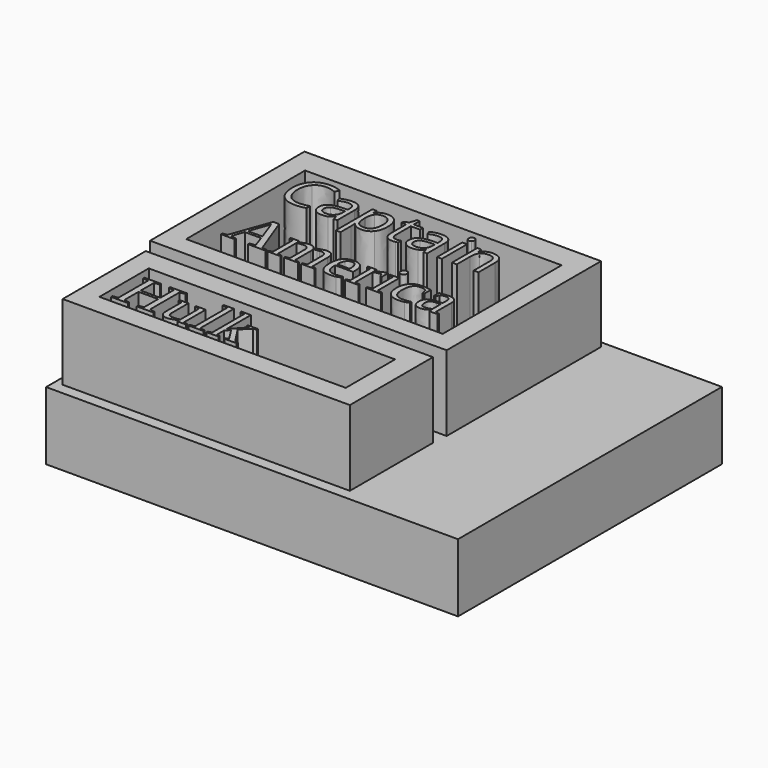
from build123d import *

# Parameters (mm, degrees)
F0_W          = 138.5813653469
F0_H          = 110.9895631671
F1_DEPTH      = 22.8698384017
F3_DEPTH      = 25.4
F4_DEPTH      = 25.4
F5_DEPTH      = 25.4
F6_DEPTH      = 25.4
F7_DEPTH      = 25.4
F2_W          = 1.612249592
F2_H          = 10.6396047259
F8_DEPTH      = 25.4
F9_DEPTH      = 25.4
F10_DEPTH     = 25.4
F11_DEPTH     = 25.4
F12_W         = 99.7868776321
F12_H         = 64.9340823293
F12_W_2       = 86.3021612167
F12_H_2       = 49.9971657991
F13_DEPTH     = 25.4
F14_W         = 96.6105125844
F14_H         = 34.9357193336
F14_W_2       = 82.8725360334
F14_H_2       = 20.7511782646
F15_DEPTH     = 25.4
F16_TEXT_SIZE = 21.4265555971
F17_DEPTH     = 25.4


# Not quite as in the source:
# - Text() gives the source's letters only with a copy of the font that has no kerning and outlines rounded to 1/6400 em; it was checked with that copy


with BuildPart() as f1:
    # F0 (on Top) → F1 (new body)
    with BuildSketch(Plane.XY):
        with Locations((2.9043704271, 4.875253886)):
            Rectangle(F0_W, F0_H)
    extrude(amount=F1_DEPTH)

    # F2 (on face) → F3 (join)
    with BuildSketch(Plane.XY.offset(22.8698384017)):
        with BuildLine():
            add(Edge.make_bspline(
                [(-49.4385806249, 46.1128756853), (-51.7777404376, 46.1128756853), (-53.1321543531, 44.5549890371)],
                knots=[0, 0, 0, 1, 1, 1], degree=2))
            add(Edge.make_bspline(
                [(-46.2140814408, 45.3580073792), (-47.8263310328, 46.1128756853), (-49.4385806249, 46.1128756853)],
                knots=[0, 0, 0, 1, 1, 1], degree=2))
            Line((-46.2140814408, 45.3580073792), (-45.5151293055, 46.7745503734))
            add(Edge.make_bspline(
                [(-49.4168354473, 47.5884413043), (-47.1864015223, 47.5884413043), (-45.5151293055, 46.7745503734)],
                knots=[0, 0, 0, 1, 1, 1], degree=2))
            add(Edge.make_bspline(
                [(-53.0622591396, 46.6953357981), (-51.5136918532, 47.5884413043), (-49.4168354473, 47.5884413043)],
                knots=[0, 0, 0, 1, 1, 1], degree=2))
            add(Edge.make_bspline(
                [(-55.4309302647, 44.1527032526), (-54.6108264259, 45.8022302919), (-53.0622591396, 46.6953357981)],
                knots=[0, 0, 0, 1, 1, 1], degree=2))
            add(Edge.make_bspline(
                [(-56.2510341034, 40.3100197355), (-56.2510341034, 42.5031762134), (-55.4309302647, 44.1527032526)],
                knots=[0, 0, 0, 1, 1, 1], degree=2))
            add(Edge.make_bspline(
                [(-54.5471441203, 34.9016834354), (-56.2510341034, 36.8059396973), (-56.2510341034, 40.3100197355)],
                knots=[0, 0, 0, 1, 1, 1], degree=2))
            add(Edge.make_bspline(
                [(-49.7088421172, 32.9974271735), (-52.8432541372, 32.9974271735), (-54.5471441203, 34.9016834354)],
                knots=[0, 0, 0, 1, 1, 1], degree=2))
            add(Edge.make_bspline(
                [(-46.0680781058, 33.5534824278), (-47.5436437248, 32.9974271735), (-49.7088421172, 32.9974271735)],
                knots=[0, 0, 0, 1, 1, 1], degree=2))
            Line((-46.0680781058, 33.5534824278), (-46.0680781058, 34.9979835074))
            add(Edge.make_bspline(
                [(-49.4572193485, 34.4636734307), (-47.9723343677, 34.4636734307), (-46.0680781058, 34.9979835074)],
                knots=[0, 0, 0, 1, 1, 1], degree=2))
            add(Edge.make_bspline(
                [(-53.1803043891, 35.9842826316), (-51.8740405096, 34.4636734307), (-49.4572193485, 34.4636734307)],
                knots=[0, 0, 0, 1, 1, 1], degree=2))
            add(Edge.make_bspline(
                [(-54.4865682686, 40.288274558), (-54.4865682686, 37.5048918326), (-53.1803043891, 35.9842826316)],
                knots=[0, 0, 0, 1, 1, 1], degree=2))
            add(Edge.make_bspline(
                [(-53.1321543531, 44.5549890371), (-54.4865682686, 42.997102389), (-54.4865682686, 40.288274558)],
                knots=[0, 0, 0, 1, 1, 1], degree=2))
        make_face()
        with BuildLine():
            add(Edge.make_bspline(
                [(-2.069186264, 20.8664472448), (-2.069186264, 20.406691862), (-2.4023423385, 20.0735357875)],
                knots=[0, 0, 0, 1, 1, 1], degree=2))
            add(Edge.make_bspline(
                [(-2.4023423385, 21.6693533843), (-2.069186264, 21.3361973098), (-2.069186264, 20.8664472448)],
                knots=[0, 0, 0, 1, 1, 1], degree=2))
            add(Edge.make_bspline(
                [(-3.2019169173, 22.0025094588), (-2.735498413, 22.0025094588), (-2.4023423385, 21.6693533843)],
                knots=[0, 0, 0, 1, 1, 1], degree=2))
            add(Edge.make_bspline(
                [(-3.9948283746, 21.6693533843), (-3.6616723001, 22.0025094588), (-3.2019169173, 22.0025094588)],
                knots=[0, 0, 0, 1, 1, 1], degree=2))
            add(Edge.make_bspline(
                [(-4.3279844491, 20.8664472448), (-4.3279844491, 21.3361973098), (-3.9948283746, 21.6693533843)],
                knots=[0, 0, 0, 1, 1, 1], degree=2))
            add(Edge.make_bspline(
                [(-3.9948283746, 20.0735357875), (-4.3279844491, 20.406691862), (-4.3279844491, 20.8664472448)],
                knots=[0, 0, 0, 1, 1, 1], degree=2))
            add(Edge.make_bspline(
                [(-3.2019169173, 19.740379713), (-3.6616723001, 19.740379713), (-3.9948283746, 20.0735357875)],
                knots=[0, 0, 0, 1, 1, 1], degree=2))
            add(Edge.make_bspline(
                [(-2.4023423385, 20.0735357875), (-2.735498413, 19.740379713), (-3.2019169173, 19.740379713)],
                knots=[0, 0, 0, 1, 1, 1], degree=2))
        make_face()
    extrude(amount=F3_DEPTH)

    # F2 (on face) → F4 (join)
    with BuildSketch(Plane.XY.offset(22.8698384017)):
        with BuildLine():
            Line((-36.991019709, 34.7090832915), (-36.6710549537, 33.1931337714))
            Line((-36.6710549537, 33.1931337714), (-35.4750701889, 33.1931337714))
            Line((-35.4750701889, 33.1931337714), (-35.4750701889, 40.4560230705))
            add(Edge.make_bspline(
                [(-36.3930273266, 43.1632976745), (-35.4750701889, 42.3198954312), (-35.4750701889, 40.4560230705)],
                knots=[0, 0, 0, 1, 1, 1], degree=2))
            add(Edge.make_bspline(
                [(-39.2121342722, 44.0066999177), (-37.3109844643, 44.0066999177), (-36.3930273266, 43.1632976745)],
                knots=[0, 0, 0, 1, 1, 1], degree=2))
            add(Edge.make_bspline(
                [(-41.0930921296, 43.7643965108), (-40.1564962683, 44.0066999177), (-39.2121342722, 44.0066999177)],
                knots=[0, 0, 0, 1, 1, 1], degree=2))
            add(Edge.make_bspline(
                [(-42.8156208363, 43.0965089149), (-42.0296879909, 43.5220931039), (-41.0930921296, 43.7643965108)],
                knots=[0, 0, 0, 1, 1, 1], degree=2))
            Line((-42.8156208363, 43.0965089149), (-42.3185882068, 41.8632467028))
            add(Edge.make_bspline(
                [(-39.3115407981, 42.6771376337), (-40.6411030821, 42.6771376337), (-42.3185882068, 41.8632467028)],
                knots=[0, 0, 0, 1, 1, 1], degree=2))
            add(Edge.make_bspline(
                [(-37.5874588644, 42.0806984783), (-38.1248753951, 42.6771376337), (-39.3115407981, 42.6771376337)],
                knots=[0, 0, 0, 1, 1, 1], degree=2))
            add(Edge.make_bspline(
                [(-37.0500423338, 40.2323583872), (-37.0500423338, 41.4842593228), (-37.5874588644, 42.0806984783)],
                knots=[0, 0, 0, 1, 1, 1], degree=2))
            Line((-37.0500423338, 40.2323583872), (-37.0500423338, 39.5706836991))
            Line((-37.0500423338, 39.5706836991), (-38.8548920697, 39.5116610744))
            add(Edge.make_bspline(
                [(-44.0084991472, 36.1349456475), (-44.0084991472, 39.3563383776), (-38.8548920697, 39.5116610744)],
                knots=[0, 0, 0, 1, 1, 1], degree=2))
            add(Edge.make_bspline(
                [(-43.1107339601, 33.8144245583), (-44.0084991472, 34.6314219431), (-44.0084991472, 36.1349456475)],
                knots=[0, 0, 0, 1, 1, 1], degree=2))
            add(Edge.make_bspline(
                [(-40.6317837203, 32.9974271735), (-42.212968773, 32.9974271735), (-43.1107339601, 33.8144245583)],
                knots=[0, 0, 0, 1, 1, 1], degree=2))
            add(Edge.make_bspline(
                [(-38.654525791, 33.3531161491), (-39.4451183173, 32.9974271735), (-40.6317837203, 32.9974271735)],
                knots=[0, 0, 0, 1, 1, 1], degree=2))
            add(Edge.make_bspline(
                [(-37.0686810574, 34.7090832915), (-37.8639332646, 33.7088051246), (-38.654525791, 33.3531161491)],
                knots=[0, 0, 0, 1, 1, 1], degree=2))
            Line((-37.0686810574, 34.7090832915), (-36.991019709, 34.7090832915))
        make_face()
        with BuildLine():
            add(Edge.make_bspline(
                [(-40.3118189651, 34.3300959115), (-38.8051888068, 34.3300959115), (-37.9462542939, 35.1548594311)],
                knots=[0, 0, 0, 1, 1, 1], degree=2))
            add(Edge.make_bspline(
                [(-41.7904910379, 34.7851914129), (-41.262393869, 34.3300959115), (-40.3118189651, 34.3300959115)],
                knots=[0, 0, 0, 1, 1, 1], degree=2))
            add(Edge.make_bspline(
                [(-42.3185882068, 36.1163069239), (-42.3185882068, 35.2402869143), (-41.7904910379, 34.7851914129)],
                knots=[0, 0, 0, 1, 1, 1], degree=2))
            add(Edge.make_bspline(
                [(-41.4705262827, 37.7611742822), (-42.3185882068, 37.2315238864), (-42.3185882068, 36.1163069239)],
                knots=[0, 0, 0, 1, 1, 1], degree=2))
            add(Edge.make_bspline(
                [(-38.699569373, 38.3591666646), (-40.6224643585, 38.2908246781), (-41.4705262827, 37.7611742822)],
                knots=[0, 0, 0, 1, 1, 1], degree=2))
            Line((-38.699569373, 38.3591666646), (-37.087319781, 38.4244021973))
            Line((-37.087319781, 38.4244021973), (-37.087319781, 37.4645079315))
            add(Edge.make_bspline(
                [(-37.9462542939, 35.1548594311), (-37.087319781, 35.9796229507), (-37.087319781, 37.4645079315)],
                knots=[0, 0, 0, 1, 1, 1], degree=2))
        make_face(mode=Mode.SUBTRACT)
    extrude(amount=F4_DEPTH)

    # F2 (on face) → F5 (join)
    with BuildSketch(Plane.XY.offset(22.8698384017)):
        with BuildLine():
            add(Edge.make_bspline(
                [(-27.2056898151, 32.9974271735), (-28.2463518832, 32.9974271735), (-29.1052863961, 33.3810742345)],
                knots=[0, 0, 0, 1, 1, 1], degree=2))
            add(Edge.make_bspline(
                [(-23.9578922265, 34.449694388), (-25.1274721328, 32.9974271735), (-27.2056898151, 32.9974271735)],
                knots=[0, 0, 0, 1, 1, 1], degree=2))
            add(Edge.make_bspline(
                [(-22.7883123201, 38.5238087232), (-22.7883123201, 35.9019616024), (-23.9578922265, 34.449694388)],
                knots=[0, 0, 0, 1, 1, 1], degree=2))
            add(Edge.make_bspline(
                [(-23.9392535029, 42.5808375617), (-22.7883123201, 41.1332300282), (-22.7883123201, 38.5238087232)],
                knots=[0, 0, 0, 1, 1, 1], degree=2))
            add(Edge.make_bspline(
                [(-27.2056898151, 44.0284450952), (-25.0901946856, 44.0284450952), (-23.9392535029, 42.5808375617)],
                knots=[0, 0, 0, 1, 1, 1], degree=2))
            add(Edge.make_bspline(
                [(-29.0990734882, 43.6401383534), (-28.2743099686, 44.0284450952), (-27.2056898151, 44.0284450952)],
                knots=[0, 0, 0, 1, 1, 1], degree=2))
            add(Edge.make_bspline(
                [(-30.5451277947, 42.375811602), (-29.9238370078, 43.2518316116), (-29.0990734882, 43.6401383534)],
                knots=[0, 0, 0, 1, 1, 1], degree=2))
            Line((-30.5451277947, 42.375811602), (-30.6227891431, 42.375811602))
            Line((-30.6227891431, 42.375811602), (-30.8464538264, 43.8327384974))
            Line((-30.8464538264, 43.8327384974), (-32.1573773868, 43.8327384974))
            Line((-32.1573773868, 43.8327384974), (-32.1573773868, 28.41540762))
            Line((-32.1573773868, 28.41540762), (-30.5451277947, 28.41540762))
            Line((-30.5451277947, 28.41540762), (-30.5451277947, 32.7955076678))
            add(Edge.make_bspline(
                [(-30.6631730443, 34.5630799566), (-30.5451277947, 33.6311437762), (-30.5451277947, 32.7955076678)],
                knots=[0, 0, 0, 1, 1, 1], degree=2))
            Line((-30.6631730443, 34.5630799566), (-30.5451277947, 34.5630799566))
            add(Edge.make_bspline(
                [(-29.1052863961, 33.3810742345), (-29.964220909, 33.7647212954), (-30.5451277947, 34.5630799566)],
                knots=[0, 0, 0, 1, 1, 1], degree=2))
        make_face()
        with BuildLine():
            add(Edge.make_bspline(
                [(-27.4386738602, 42.6584989101), (-29.0695621758, 42.6584989101), (-29.7980256235, 41.7560740421)],
                knots=[0, 0, 0, 1, 1, 1], degree=2))
            add(Edge.make_bspline(
                [(-25.2408577014, 41.5960916645), (-26.022130866, 42.6584989101), (-27.4386738602, 42.6584989101)],
                knots=[0, 0, 0, 1, 1, 1], degree=2))
            add(Edge.make_bspline(
                [(-24.4595845369, 38.5424474468), (-24.4595845369, 40.5336844188), (-25.2408577014, 41.5960916645)],
                knots=[0, 0, 0, 1, 1, 1], degree=2))
            add(Edge.make_bspline(
                [(-25.2408577014, 35.4655048246), (-24.4595845369, 36.582275014), (-24.4595845369, 38.5424474468)],
                knots=[0, 0, 0, 1, 1, 1], degree=2))
            add(Edge.make_bspline(
                [(-27.4013964129, 34.3487346351), (-26.022130866, 34.3487346351), (-25.2408577014, 35.4655048246)],
                knots=[0, 0, 0, 1, 1, 1], degree=2))
            add(Edge.make_bspline(
                [(-29.7980256235, 35.3148418087), (-29.0509234522, 34.3487346351), (-27.4013964129, 34.3487346351)],
                knots=[0, 0, 0, 1, 1, 1], degree=2))
            add(Edge.make_bspline(
                [(-30.5451277947, 38.5238087232), (-30.5451277947, 36.2809489824), (-29.7980256235, 35.3148418087)],
                knots=[0, 0, 0, 1, 1, 1], degree=2))
            Line((-30.5451277947, 38.5238087232), (-30.5451277947, 38.8810509256))
            add(Edge.make_bspline(
                [(-29.7980256235, 41.7560740421), (-30.5264890711, 40.8536491741), (-30.5451277947, 38.8810509256)],
                knots=[0, 0, 0, 1, 1, 1], degree=2))
        make_face(mode=Mode.SUBTRACT)
    extrude(amount=F5_DEPTH)

    # F2 (on face) → F6 (join)
    with BuildSketch(Plane.XY.offset(22.8698384017)):
        with BuildLine():
            add(Edge.make_bspline(
                [(-16.5381270037, 34.3300959115), (-16.1094363607, 34.3300959115), (-15.7118102571, 34.3922249902)],
                knots=[0, 0, 0, 1, 1, 1], degree=2))
            add(Edge.make_bspline(
                [(-17.7900279394, 34.8442140376), (-17.333379211, 34.3300959115), (-16.5381270037, 34.3300959115)],
                knots=[0, 0, 0, 1, 1, 1], degree=2))
            add(Edge.make_bspline(
                [(-18.2466766677, 36.3182264296), (-18.2466766677, 35.3583321638), (-17.7900279394, 34.8442140376)],
                knots=[0, 0, 0, 1, 1, 1], degree=2))
            Line((-18.2466766677, 36.3182264296), (-18.2466766677, 42.5808375617))
            Line((-18.2466766677, 42.5808375617), (-15.1588614568, 42.5808375617))
            Line((-15.1588614568, 42.5808375617), (-15.1588614568, 43.8327384974))
            Line((-15.1588614568, 43.8327384974), (-18.2466766677, 43.8327384974))
            Line((-18.2466766677, 43.8327384974), (-18.2466766677, 46.2992629214))
            Line((-18.2466766677, 46.2992629214), (-19.1786128481, 46.2992629214))
            Line((-19.1786128481, 46.2992629214), (-19.8558198058, 44.0284450952))
            Line((-19.8558198058, 44.0284450952), (-21.3810886877, 43.3574510454))
            Line((-21.3810886877, 43.3574510454), (-21.3810886877, 42.5808375617))
            Line((-21.3810886877, 42.5808375617), (-19.8558198058, 42.5808375617))
            Line((-19.8558198058, 42.5808375617), (-19.8558198058, 36.249884443))
            add(Edge.make_bspline(
                [(-16.7711110488, 32.9974271735), (-19.8558198058, 32.9974271735), (-19.8558198058, 36.249884443)],
                knots=[0, 0, 0, 1, 1, 1], degree=2))
            add(Edge.make_bspline(
                [(-15.8516006842, 33.0813014298), (-16.3610591294, 32.9974271735), (-16.7711110488, 32.9974271735)],
                knots=[0, 0, 0, 1, 1, 1], degree=2))
            add(Edge.make_bspline(
                [(-15.0812001084, 33.2894338434), (-15.3421422389, 33.165175686), (-15.8516006842, 33.0813014298)],
                knots=[0, 0, 0, 1, 1, 1], degree=2))
            Line((-15.0812001084, 33.2894338434), (-15.0812001084, 34.5226960554))
            add(Edge.make_bspline(
                [(-15.7118102571, 34.3922249902), (-15.3141841535, 34.4543540689), (-15.0812001084, 34.5226960554)],
                knots=[0, 0, 0, 1, 1, 1], degree=2))
        make_face()
    extrude(amount=F6_DEPTH)

    # F2 (on face) → F7 (join)
    with BuildSketch(Plane.XY.offset(22.8698384017)):
        with BuildLine():
            Line((-6.7341583862, 34.7090832915), (-6.4141936309, 33.1931337714))
            Line((-6.4141936309, 33.1931337714), (-5.2182088661, 33.1931337714))
            Line((-5.2182088661, 33.1931337714), (-5.2182088661, 40.4560230705))
            add(Edge.make_bspline(
                [(-6.1361660038, 43.1632976745), (-5.2182088661, 42.3198954312), (-5.2182088661, 40.4560230705)],
                knots=[0, 0, 0, 1, 1, 1], degree=2))
            add(Edge.make_bspline(
                [(-8.9552729494, 44.0066999177), (-7.0541231414, 44.0066999177), (-6.1361660038, 43.1632976745)],
                knots=[0, 0, 0, 1, 1, 1], degree=2))
            add(Edge.make_bspline(
                [(-10.8362308068, 43.7643965108), (-9.8996349455, 44.0066999177), (-8.9552729494, 44.0066999177)],
                knots=[0, 0, 0, 1, 1, 1], degree=2))
            add(Edge.make_bspline(
                [(-12.5587595135, 43.0965089149), (-11.7728266681, 43.5220931039), (-10.8362308068, 43.7643965108)],
                knots=[0, 0, 0, 1, 1, 1], degree=2))
            Line((-12.5587595135, 43.0965089149), (-12.061726884, 41.8632467028))
            add(Edge.make_bspline(
                [(-9.0546794753, 42.6771376337), (-10.3842417593, 42.6771376337), (-12.061726884, 41.8632467028)],
                knots=[0, 0, 0, 1, 1, 1], degree=2))
            add(Edge.make_bspline(
                [(-7.3305975416, 42.0806984783), (-7.8680140723, 42.6771376337), (-9.0546794753, 42.6771376337)],
                knots=[0, 0, 0, 1, 1, 1], degree=2))
            add(Edge.make_bspline(
                [(-6.7931810109, 40.2323583872), (-6.7931810109, 41.4842593228), (-7.3305975416, 42.0806984783)],
                knots=[0, 0, 0, 1, 1, 1], degree=2))
            Line((-6.7931810109, 40.2323583872), (-6.7931810109, 39.5706836991))
            Line((-6.7931810109, 39.5706836991), (-8.5980307469, 39.5116610744))
            add(Edge.make_bspline(
                [(-13.7516378244, 36.1349456475), (-13.7516378244, 39.3563383776), (-8.5980307469, 39.5116610744)],
                knots=[0, 0, 0, 1, 1, 1], degree=2))
            add(Edge.make_bspline(
                [(-12.8538726373, 33.8144245583), (-13.7516378244, 34.6314219431), (-13.7516378244, 36.1349456475)],
                knots=[0, 0, 0, 1, 1, 1], degree=2))
            add(Edge.make_bspline(
                [(-10.3749223975, 32.9974271735), (-11.9561074502, 32.9974271735), (-12.8538726373, 33.8144245583)],
                knots=[0, 0, 0, 1, 1, 1], degree=2))
            add(Edge.make_bspline(
                [(-8.3976644681, 33.3531161491), (-9.1882569945, 32.9974271735), (-10.3749223975, 32.9974271735)],
                knots=[0, 0, 0, 1, 1, 1], degree=2))
            add(Edge.make_bspline(
                [(-6.8118197345, 34.7090832915), (-7.6070719418, 33.7088051246), (-8.3976644681, 33.3531161491)],
                knots=[0, 0, 0, 1, 1, 1], degree=2))
            Line((-6.8118197345, 34.7090832915), (-6.7341583862, 34.7090832915))
        make_face()
        with BuildLine():
            add(Edge.make_bspline(
                [(-10.0549576422, 34.3300959115), (-8.548327484, 34.3300959115), (-7.6893929711, 35.1548594311)],
                knots=[0, 0, 0, 1, 1, 1], degree=2))
            add(Edge.make_bspline(
                [(-11.5336297151, 34.7851914129), (-11.0055325462, 34.3300959115), (-10.0549576422, 34.3300959115)],
                knots=[0, 0, 0, 1, 1, 1], degree=2))
            add(Edge.make_bspline(
                [(-12.061726884, 36.1163069239), (-12.061726884, 35.2402869143), (-11.5336297151, 34.7851914129)],
                knots=[0, 0, 0, 1, 1, 1], degree=2))
            add(Edge.make_bspline(
                [(-11.2136649598, 37.7611742822), (-12.061726884, 37.2315238864), (-12.061726884, 36.1163069239)],
                knots=[0, 0, 0, 1, 1, 1], degree=2))
            add(Edge.make_bspline(
                [(-8.4427080502, 38.3591666646), (-10.3656030357, 38.2908246781), (-11.2136649598, 37.7611742822)],
                knots=[0, 0, 0, 1, 1, 1], degree=2))
            Line((-8.4427080502, 38.3591666646), (-6.8304584582, 38.4244021973))
            Line((-6.8304584582, 38.4244021973), (-6.8304584582, 37.4645079315))
            add(Edge.make_bspline(
                [(-7.6893929711, 35.1548594311), (-6.8304584582, 35.9796229507), (-6.8304584582, 37.4645079315)],
                knots=[0, 0, 0, 1, 1, 1], degree=2))
        make_face(mode=Mode.SUBTRACT)
    extrude(amount=F7_DEPTH)

    # F2 (on face) → F8 (join)
    with BuildSketch(Plane.XY.offset(22.8698384017)):
        with BuildLine():
            add(Edge.make_bspline(
                [(-2.0372000371, 46.7155277487), (-2.0372000371, 47.268476549), (-1.7653853178, 47.5263122256)],
                knots=[0, 0, 0, 1, 1, 1], degree=2))
            add(Edge.make_bspline(
                [(-1.7653853178, 45.9047432717), (-2.0372000371, 46.1718983101), (-2.0372000371, 46.7155277487)],
                knots=[0, 0, 0, 1, 1, 1], degree=2))
            add(Edge.make_bspline(
                [(-1.0835186792, 45.6375882334), (-1.4935705985, 45.6375882334), (-1.7653853178, 45.9047432717)],
                knots=[0, 0, 0, 1, 1, 1], degree=2))
            add(Edge.make_bspline(
                [(-0.4140778563, 45.9047432717), (-0.6952119374, 45.6375882334), (-1.0835186792, 45.6375882334)],
                knots=[0, 0, 0, 1, 1, 1], degree=2))
            add(Edge.make_bspline(
                [(-0.1329437752, 46.7155277487), (-0.1329437752, 46.1718983101), (-0.4140778563, 45.9047432717)],
                knots=[0, 0, 0, 1, 1, 1], degree=2))
            add(Edge.make_bspline(
                [(-0.4140778563, 47.5216525447), (-0.1329437752, 47.2591571872), (-0.1329437752, 46.7155277487)],
                knots=[0, 0, 0, 1, 1, 1], degree=2))
            add(Edge.make_bspline(
                [(-1.0835186792, 47.7841479021), (-0.6952119374, 47.7841479021), (-0.4140778563, 47.5216525447)],
                knots=[0, 0, 0, 1, 1, 1], degree=2))
            add(Edge.make_bspline(
                [(-1.7653853178, 47.5263122256), (-1.4935705985, 47.7841479021), (-1.0835186792, 47.7841479021)],
                knots=[0, 0, 0, 1, 1, 1], degree=2))
        make_face()
        with Locations((-1.0943912679, 38.5129361344)):
            Rectangle(F2_W, F2_H)
    extrude(amount=F8_DEPTH)

    # F2 (on face) → F9 (join)
    with BuildSketch(Plane.XY.offset(22.8698384017)):
        with BuildLine():
            Line((10.4103608788, 40.0770356905), (10.4103608788, 33.1931337714))
            Line((10.4103608788, 33.1931337714), (12.0226104708, 33.1931337714))
            Line((12.0226104708, 33.1931337714), (12.0226104708, 40.1329518613))
            add(Edge.make_bspline(
                [(11.0518436163, 43.1011685958), (12.0226104708, 42.1738920963), (12.0226104708, 40.1329518613)],
                knots=[0, 0, 0, 1, 1, 1], degree=2))
            add(Edge.make_bspline(
                [(8.1581817762, 44.0284450952), (10.0810767617, 44.0284450952), (11.0518436163, 43.1011685958)],
                knots=[0, 0, 0, 1, 1, 1], degree=2))
            add(Edge.make_bspline(
                [(6.1684980311, 43.5950947714), (7.0616035373, 44.0284450952), (8.1581817762, 44.0284450952)],
                knots=[0, 0, 0, 1, 1, 1], degree=2))
            add(Edge.make_bspline(
                [(4.7783598954, 42.375811602), (5.2753925249, 43.1617444475), (6.1684980311, 43.5950947714)],
                knots=[0, 0, 0, 1, 1, 1], degree=2))
            Line((4.7783598954, 42.375811602), (4.700698547, 42.375811602))
            Line((4.700698547, 42.375811602), (4.4397564165, 43.8327384974))
            Line((4.4397564165, 43.8327384974), (3.1288328561, 43.8327384974))
            Line((3.1288328561, 43.8327384974), (3.1288328561, 33.1931337714))
            Line((3.1288328561, 33.1931337714), (4.7410824482, 33.1931337714))
            Line((4.7410824482, 33.1931337714), (4.7410824482, 38.7754314919))
            add(Edge.make_bspline(
                [(5.5176959318, 41.7560740421), (4.7410824482, 40.8536491741), (4.7410824482, 38.7754314919)],
                knots=[0, 0, 0, 1, 1, 1], degree=2))
            add(Edge.make_bspline(
                [(7.9624751783, 42.6584989101), (6.2943094155, 42.6584989101), (5.5176959318, 41.7560740421)],
                knots=[0, 0, 0, 1, 1, 1], degree=2))
            add(Edge.make_bspline(
                [(9.8185814042, 42.0170161726), (9.2268019297, 42.6584989101), (7.9624751783, 42.6584989101)],
                knots=[0, 0, 0, 1, 1, 1], degree=2))
            add(Edge.make_bspline(
                [(10.4103608788, 40.0770356905), (10.4103608788, 41.3755334351), (9.8185814042, 42.0170161726)],
                knots=[0, 0, 0, 1, 1, 1], degree=2))
        make_face()
    extrude(amount=F9_DEPTH)

    # F2 (on face) → F10 (join)
    with BuildSketch(Plane.XY.offset(22.8698384017)):
        Polygon((-49.7604783288, 7.8833550215), (-49.7604783288, 8.4363941051), (-51.6361470282, 8.7162452077), (-50.2302283939, 12.7441021484), (-44.7331531646, 12.7441021484), (-43.3472238947, 8.7162452077), (-45.2228925941, 8.4363941051), (-45.2228925941, 7.8833550215), (-39.319366954, 7.8833550215), (-39.319366954, 8.4363941051), (-41.0884257096, 8.7162452077), (-46.0357934159, 21.9591991691), (-48.0114089377, 21.9591991691), (-52.7688776816, 8.7162452077), (-54.3513690354, 8.4363941051), (-54.3513690354, 7.8833550215), align=None)
        Polygon((-49.9170616838, 13.6836022785), (-47.5216695082, 20.4599968339), (-45.0563145569, 13.6836022785), align=None, mode=Mode.SUBTRACT)
        with BuildLine():
            add(Edge.make_bspline(
                [(-35.7679231998, 16.878569033), (-34.9883379854, 17.3249981728), (-34.1138032899, 17.6281702006)],
                knots=[0, 0, 0, 1, 1, 1], degree=2))
            Line((-35.7679231998, 16.878569033), (-35.8512122184, 17.6714804903))
            Line((-35.8512122184, 17.6714804903), (-38.7163544591, 17.6714804903))
            Line((-38.7163544591, 17.6714804903), (-38.7163544591, 17.2017304253))
            Line((-38.7163544591, 17.2017304253), (-37.477013862, 16.9418686872))
            Line((-37.477013862, 16.9418686872), (-37.477013862, 8.6129668246))
            Line((-37.477013862, 8.6129668246), (-38.7163544591, 8.3531050865))
            Line((-38.7163544591, 8.3531050865), (-38.7163544591, 7.8833550215))
            Line((-38.7163544591, 7.8833550215), (-34.2787155468, 7.8833550215))
            Line((-34.2787155468, 7.8833550215), (-34.2787155468, 8.3531050865))
            Line((-34.2787155468, 8.3531050865), (-35.7479338353, 8.6129668246))
            Line((-35.7479338353, 8.6129668246), (-35.7479338353, 16.3488508745))
            add(Edge.make_bspline(
                [(-33.4691462857, 16.6486913416), (-34.3853254906, 16.6486913416), (-35.7479338353, 16.3488508745)],
                knots=[0, 0, 0, 1, 1, 1], degree=2))
            add(Edge.make_bspline(
                [(-32.1398535485, 16.185604398), (-32.5829511276, 16.6486913416), (-33.4691462857, 16.6486913416)],
                knots=[0, 0, 0, 1, 1, 1], degree=2))
            add(Edge.make_bspline(
                [(-31.6967559694, 14.8596432215), (-31.6967559694, 15.7225174545), (-32.1398535485, 16.185604398)],
                knots=[0, 0, 0, 1, 1, 1], degree=2))
            Line((-31.6967559694, 14.8596432215), (-31.6967559694, 8.6129668246))
            Line((-31.6967559694, 8.6129668246), (-33.1459848935, 8.3531050865))
            Line((-33.1459848935, 8.3531050865), (-33.1459848935, 7.8833550215))
            Line((-33.1459848935, 7.8833550215), (-28.5017892149, 7.8833550215))
            Line((-28.5017892149, 7.8833550215), (-28.5017892149, 8.3531050865))
            Line((-28.5017892149, 8.3531050865), (-29.9710075035, 8.6129668246))
            Line((-29.9710075035, 8.6129668246), (-29.9710075035, 15.0462106232))
            add(Edge.make_bspline(
                [(-30.147580223, 16.2855512204), (-29.9710075035, 15.7225174545), (-29.9710075035, 15.0462106232)],
                knots=[0, 0, 0, 1, 1, 1], degree=2))
            add(Edge.make_bspline(
                [(-29.5995384804, 16.3938269446), (-29.9276972138, 16.3255299493), (-30.147580223, 16.2855512204)],
                knots=[0, 0, 0, 1, 1, 1], degree=2))
            add(Edge.make_bspline(
                [(-28.9132369669, 16.5137631314), (-29.271379747, 16.4621239399), (-29.5995384804, 16.3938269446)],
                knots=[0, 0, 0, 1, 1, 1], degree=2))
            add(Edge.make_bspline(
                [(-28.1952856264, 16.6070468323), (-28.5550941868, 16.565402323), (-28.9132369669, 16.5137631314)],
                knots=[0, 0, 0, 1, 1, 1], degree=2))
            add(Edge.make_bspline(
                [(-27.5656206456, 16.6486913416), (-27.8354770659, 16.6486913416), (-28.1952856264, 16.6070468323)],
                knots=[0, 0, 0, 1, 1, 1], degree=2))
            add(Edge.make_bspline(
                [(-25.8998402731, 14.8596432215), (-25.8998402731, 16.6486913416), (-27.5656206456, 16.6486913416)],
                knots=[0, 0, 0, 1, 1, 1], degree=2))
            Line((-25.8998402731, 14.8596432215), (-25.8998402731, 8.6129668246))
            Line((-25.8998402731, 8.6129668246), (-27.3557323186, 8.3531050865))
            Line((-27.3557323186, 8.3531050865), (-27.3557323186, 7.8833550215))
            Line((-27.3557323186, 7.8833550215), (-22.9114302848, 7.8833550215))
            Line((-22.9114302848, 7.8833550215), (-22.9114302848, 8.3531050865))
            Line((-22.9114302848, 8.3531050865), (-24.1707602464, 8.6129668246))
            Line((-24.1707602464, 8.6129668246), (-24.1707602464, 15.0462106232))
            add(Edge.make_bspline(
                [(-26.6694308052, 17.9313422284), (-24.1707602464, 17.9313422284), (-24.1707602464, 15.0462106232)],
                knots=[0, 0, 0, 1, 1, 1], degree=2))
            add(Edge.make_bspline(
                [(-28.4534815841, 17.5865256913), (-27.3757216831, 17.9313422284), (-26.6694308052, 17.9313422284)],
                knots=[0, 0, 0, 1, 1, 1], degree=2))
            add(Edge.make_bspline(
                [(-30.3341476247, 16.7952800144), (-29.5312414851, 17.2417091542), (-28.4534815841, 17.5865256913)],
                knots=[0, 0, 0, 1, 1, 1], degree=2))
            add(Edge.make_bspline(
                [(-31.2453294884, 17.6598200277), (-30.6373196525, 17.388297827), (-30.3341476247, 16.7952800144)],
                knots=[0, 0, 0, 1, 1, 1], degree=2))
            add(Edge.make_bspline(
                [(-32.5729564453, 17.9313422284), (-31.8533393244, 17.9313422284), (-31.2453294884, 17.6598200277)],
                knots=[0, 0, 0, 1, 1, 1], degree=2))
            add(Edge.make_bspline(
                [(-34.1138032899, 17.6281702006), (-33.2392685943, 17.9313422284), (-32.5729564453, 17.9313422284)],
                knots=[0, 0, 0, 1, 1, 1], degree=2))
        make_face()
        with BuildLine():
            Line((-19.8697153246, 12.6208344009), (-19.8697153246, 12.8074018026))
            Line((-19.8697153246, 12.8074018026), (-13.8529166191, 12.8074018026))
            Line((-13.8529166191, 12.8074018026), (-13.8529166191, 13.6602813533))
            add(Edge.make_bspline(
                [(-17.6109171395, 17.9313422284), (-13.8529166191, 17.9313422284), (-13.8529166191, 13.6602813533)],
                knots=[0, 0, 0, 1, 1, 1], degree=2))
            add(Edge.make_bspline(
                [(-20.6726214641, 16.6703464864), (-19.5998589043, 17.9313422284), (-17.6109171395, 17.9313422284)],
                knots=[0, 0, 0, 1, 1, 1], degree=2))
            add(Edge.make_bspline(
                [(-21.745384024, 12.8507120923), (-21.745384024, 15.4093507444), (-20.6726214641, 16.6703464864)],
                knots=[0, 0, 0, 1, 1, 1], degree=2))
            add(Edge.make_bspline(
                [(-20.6892792679, 8.9028126094), (-21.745384024, 10.1321585244), (-21.745384024, 12.8507120923)],
                knots=[0, 0, 0, 1, 1, 1], degree=2))
            add(Edge.make_bspline(
                [(-17.3510554014, 7.6734666945), (-19.6331745117, 7.6734666945), (-20.6892792679, 8.9028126094)],
                knots=[0, 0, 0, 1, 1, 1], degree=2))
            add(Edge.make_bspline(
                [(-15.5969886691, 7.9133390682), (-16.454865561, 7.6734666945), (-17.3510554014, 7.6734666945)],
                knots=[0, 0, 0, 1, 1, 1], degree=2))
            add(Edge.make_bspline(
                [(-14.2393776655, 8.4763728341), (-14.7391117773, 8.1532114418), (-15.5969886691, 7.9133390682)],
                knots=[0, 0, 0, 1, 1, 1], degree=2))
            Line((-14.2393776655, 8.4763728341), (-14.2393776655, 9.0593959645))
            add(Edge.make_bspline(
                [(-15.5087023094, 8.8528391983), (-14.7391117773, 8.9461228991), (-14.2393776655, 9.0593959645)],
                knots=[0, 0, 0, 1, 1, 1], degree=2))
            add(Edge.make_bspline(
                [(-16.8413266074, 8.7595554974), (-16.2782928415, 8.7595554974), (-15.5087023094, 8.8528391983)],
                knots=[0, 0, 0, 1, 1, 1], degree=2))
            add(Edge.make_bspline(
                [(-18.5754039752, 9.1760005905), (-17.9140891673, 8.7595554974), (-16.8413266074, 8.7595554974)],
                knots=[0, 0, 0, 1, 1, 1], degree=2))
            add(Edge.make_bspline(
                [(-19.5532170538, 10.3886887017), (-19.2367187831, 9.5924456837), (-18.5754039752, 9.1760005905)],
                knots=[0, 0, 0, 1, 1, 1], degree=2))
            add(Edge.make_bspline(
                [(-19.8697153246, 12.6208344009), (-19.8697153246, 11.1849317198), (-19.5532170538, 10.3886887017)],
                knots=[0, 0, 0, 1, 1, 1], degree=2))
        make_face()
        with BuildLine():
            add(Edge.make_bspline(
                [(-17.6109171395, 17.0984520422), (-18.6936743816, 17.0984520422), (-19.2717001709, 16.2239173466)],
                knots=[0, 0, 0, 1, 1, 1], degree=2))
            add(Edge.make_bspline(
                [(-16.1433646313, 16.3022090241), (-16.6214435982, 17.0984520422), (-17.6109171395, 17.0984520422)],
                knots=[0, 0, 0, 1, 1, 1], degree=2))
            add(Edge.make_bspline(
                [(-15.6652856644, 13.6402919888), (-15.6652856644, 15.5059660061), (-16.1433646313, 16.3022090241)],
                knots=[0, 0, 0, 1, 1, 1], degree=2))
            Line((-15.6652856644, 13.6402919888), (-19.8497259601, 13.6402919888))
            add(Edge.make_bspline(
                [(-19.2717001709, 16.2239173466), (-19.8497259601, 15.349382651), (-19.8497259601, 13.6402919888)],
                knots=[0, 0, 0, 1, 1, 1], degree=2))
        make_face(mode=Mode.SUBTRACT)
        with BuildLine():
            Line((-6.2003215878, 15.2860829969), (-6.2003215878, 17.9313422284))
            Line((-6.2003215878, 17.9313422284), (-6.3569049429, 17.9313422284))
            add(Edge.make_bspline(
                [(-8.0476720209, 17.4515974811), (-6.9799068022, 17.9313422284), (-6.3569049429, 17.9313422284)],
                knots=[0, 0, 0, 1, 1, 1], degree=2))
            add(Edge.make_bspline(
                [(-9.738439099, 16.4521292576), (-9.1154372397, 16.9718527339), (-8.0476720209, 17.4515974811)],
                knots=[0, 0, 0, 1, 1, 1], degree=2))
            Line((-9.738439099, 16.4521292576), (-9.8350543606, 17.6714804903))
            Line((-9.8350543606, 17.6714804903), (-12.6868703584, 17.6714804903))
            Line((-12.6868703584, 17.6714804903), (-12.6868703584, 17.2017304253))
            Line((-12.6868703584, 17.2017304253), (-11.4475297612, 16.9418686872))
            Line((-11.4475297612, 16.9418686872), (-11.4475297612, 8.6129668246))
            Line((-11.4475297612, 8.6129668246), (-12.6868703584, 8.3531050865))
            Line((-12.6868703584, 8.3531050865), (-12.6868703584, 7.8833550215))
            Line((-12.6868703584, 7.8833550215), (-8.0426746798, 7.8833550215))
            Line((-8.0426746798, 7.8833550215), (-8.0426746798, 8.3531050865))
            Line((-8.0426746798, 8.3531050865), (-9.7184497346, 8.6129668246))
            Line((-9.7184497346, 8.6129668246), (-9.7184497346, 15.9224110992))
            add(Edge.make_bspline(
                [(-8.4857722589, 16.2905485615), (-9.1987262583, 16.1489572298), (-9.7184497346, 15.9224110992)],
                knots=[0, 0, 0, 1, 1, 1], degree=2))
            add(Edge.make_bspline(
                [(-7.2530947833, 16.4321398932), (-7.7728182595, 16.4321398932), (-8.4857722589, 16.2905485615)],
                knots=[0, 0, 0, 1, 1, 1], degree=2))
            Line((-7.2530947833, 16.4321398932), (-6.6467507277, 15.2860829969))
            Line((-6.6467507277, 15.2860829969), (-6.2003215878, 15.2860829969))
        make_face()
        Polygon((-0.4966895924, 8.3531050865), (-2.1724646471, 8.6129668246), (-2.1724646471, 17.6714804903), (-5.284142383, 17.6714804903), (-5.284142383, 17.2017304253), (-3.9015446738, 16.9418686872), (-3.9015446738, 8.6129668246), (-5.5673250463, 8.3531050865), (-5.5673250463, 7.8833550215), (-0.4966895924, 7.8833550215), align=None)
    extrude(amount=F10_DEPTH)

    # F2 (on face) → F11 (join)
    with BuildSketch(Plane.XY.offset(22.8698384017)):
        Polygon((-0.4966895924, 8.3531050865), (-2.1724646471, 8.6129668246), (-2.1724646471, 17.6714804903), (-5.284142383, 17.6714804903), (-5.284142383, 17.2017304253), (-3.9015446738, 16.9418686872), (-3.9015446738, 8.6129668246), (-5.5673250463, 8.3531050865), (-5.5673250463, 7.8833550215), (-0.4966895924, 7.8833550215), align=None)
        with BuildLine():
            add(Edge.make_bspline(
                [(8.7184074283, 8.4763728341), (8.2086786343, 8.1032380306), (7.3124887939, 7.8883523626)],
                knots=[0, 0, 0, 1, 1, 1], degree=2))
            Line((8.7184074283, 8.4763728341), (8.7184074283, 9.1027062541))
            add(Edge.make_bspline(
                [(6.0731481968, 8.7595554974), (7.5923398965, 8.7595554974), (8.7184074283, 9.1027062541)],
                knots=[0, 0, 0, 1, 1, 1], degree=2))
            add(Edge.make_bspline(
                [(3.444546769, 9.7007214079), (4.2940947589, 8.7595554974), (6.0731481968, 8.7595554974)],
                knots=[0, 0, 0, 1, 1, 1], degree=2))
            add(Edge.make_bspline(
                [(2.594998779, 12.8507120923), (2.594998779, 10.6418873183), (3.444546769, 9.7007214079)],
                knots=[0, 0, 0, 1, 1, 1], degree=2))
            add(Edge.make_bspline(
                [(5.3868466833, 17.0984520422), (2.594998779, 17.0984520422), (2.594998779, 12.8507120923)],
                knots=[0, 0, 0, 1, 1, 1], degree=2))
            add(Edge.make_bspline(
                [(7.4590774667, 16.6087126127), (6.592871673, 17.0984520422), (5.3868466833, 17.0984520422)],
                knots=[0, 0, 0, 1, 1, 1], degree=2))
            Line((7.4590774667, 16.6087126127), (7.9055066065, 14.879632586))
            Line((7.9055066065, 14.879632586), (8.4785350547, 14.879632586))
            Line((8.4785350547, 14.879632586), (8.4785350547, 17.6081808362))
            add(Edge.make_bspline(
                [(5.4068360478, 17.9313422284), (6.8127546822, 17.9313422284), (8.4785350547, 17.6081808362)],
                knots=[0, 0, 0, 1, 1, 1], degree=2))
            add(Edge.make_bspline(
                [(1.9353497515, 16.6137099538), (3.1480378627, 17.9313422284), (5.4068360478, 17.9313422284)],
                knots=[0, 0, 0, 1, 1, 1], degree=2))
            add(Edge.make_bspline(
                [(0.7226616403, 12.8507120923), (0.7226616403, 15.2960776791), (1.9353497515, 16.6137099538)],
                knots=[0, 0, 0, 1, 1, 1], degree=2))
            add(Edge.make_bspline(
                [(5.4801303842, 7.6734666945), (0.7226616403, 7.6734666945), (0.7226616403, 12.8507120923)],
                knots=[0, 0, 0, 1, 1, 1], degree=2))
            add(Edge.make_bspline(
                [(7.3124887939, 7.8883523626), (6.4162989535, 7.6734666945), (5.4801303842, 7.6734666945)],
                knots=[0, 0, 0, 1, 1, 1], degree=2))
        make_face()
        with BuildLine():
            add(Edge.make_bspline(
                [(14.2154826576, 17.8880319387), (15.8179633759, 17.8880319387), (16.574227665, 17.231714472)],
                knots=[0, 0, 0, 1, 1, 1], degree=2))
            add(Edge.make_bspline(
                [(11.2503935945, 17.5248918175), (12.9361633315, 17.8880319387), (14.2154826576, 17.8880319387)],
                knots=[0, 0, 0, 1, 1, 1], degree=2))
            Line((11.2503935945, 17.5248918175), (11.2503935945, 15.38936138))
            Line((11.2503935945, 15.38936138), (11.8334167249, 15.38936138))
            Line((11.8334167249, 15.38936138), (12.1865621639, 16.6087126127))
            add(Edge.make_bspline(
                [(14.09221491, 17.0984520422), (13.0494363968, 17.0984520422), (12.1865621639, 16.6087126127)],
                knots=[0, 0, 0, 1, 1, 1], degree=2))
            add(Edge.make_bspline(
                [(15.2316086848, 16.6187072949), (14.8618054421, 17.0984520422), (14.09221491, 17.0984520422)],
                knots=[0, 0, 0, 1, 1, 1], degree=2))
            add(Edge.make_bspline(
                [(15.6014119275, 15.1294996419), (15.6014119275, 16.1389625476), (15.2316086848, 16.6187072949)],
                knots=[0, 0, 0, 1, 1, 1], degree=2))
            Line((15.6014119275, 15.1294996419), (15.6014119275, 13.6003132599))
            Line((15.6014119275, 13.6003132599), (14.1321936389, 13.5570029702))
            add(Edge.make_bspline(
                [(11.7168120988, 13.1888655079), (12.5497022851, 13.5270189235), (14.1321936389, 13.5570029702)],
                knots=[0, 0, 0, 1, 1, 1], degree=2))
            add(Edge.make_bspline(
                [(10.5041239876, 12.2093866489), (10.8839219126, 12.8507120923), (11.7168120988, 13.1888655079)],
                knots=[0, 0, 0, 1, 1, 1], degree=2))
            add(Edge.make_bspline(
                [(10.1243260627, 10.5919139072), (10.1243260627, 11.5680612055), (10.5041239876, 12.2093866489)],
                knots=[0, 0, 0, 1, 1, 1], degree=2))
            add(Edge.make_bspline(
                [(12.6329913037, 7.6734666945), (10.1243260627, 7.6734666945), (10.1243260627, 10.5919139072)],
                knots=[0, 0, 0, 1, 1, 1], degree=2))
            add(Edge.make_bspline(
                [(15.6647115816, 8.8628338805), (14.4753443957, 7.6734666945), (12.6329913037, 7.6734666945)],
                knots=[0, 0, 0, 1, 1, 1], degree=2))
            Line((15.6647115816, 8.8628338805), (15.8612736656, 7.8833550215))
            Line((15.8612736656, 7.8833550215), (18.5465116261, 7.8833550215))
            Line((18.5465116261, 7.8833550215), (18.5465116261, 8.3531050865))
            Line((18.5465116261, 8.3531050865), (17.3304919542, 8.6129668246))
            Line((17.3304919542, 8.6129668246), (17.3304919542, 15.2227833427))
            add(Edge.make_bspline(
                [(16.574227665, 17.231714472), (17.3304919542, 16.5753970052), (17.3304919542, 15.2227833427)],
                knots=[0, 0, 0, 1, 1, 1], degree=2))
        make_face()
        with BuildLine():
            Line((14.235472022, 12.8273911671), (15.6014119275, 12.8707014568))
            Line((15.6014119275, 12.8707014568), (15.6014119275, 9.392552039))
            add(Edge.make_bspline(
                [(14.5652965358, 8.981104287), (15.0816884513, 9.1426849831), (15.6014119275, 9.392552039)],
                knots=[0, 0, 0, 1, 1, 1], degree=2))
            add(Edge.make_bspline(
                [(13.3426137424, 8.8195235908), (14.0489046203, 8.8195235908), (14.5652965358, 8.981104287)],
                knots=[0, 0, 0, 1, 1, 1], degree=2))
            add(Edge.make_bspline(
                [(11.8534060894, 10.6518820006), (11.8534060894, 8.8195235908), (13.3426137424, 8.8195235908)],
                knots=[0, 0, 0, 1, 1, 1], degree=2))
            add(Edge.make_bspline(
                [(12.34814286, 12.2876783264), (11.8534060894, 11.7979388969), (11.8534060894, 10.6518820006)],
                knots=[0, 0, 0, 1, 1, 1], degree=2))
            add(Edge.make_bspline(
                [(14.235472022, 12.8273911671), (12.8428796306, 12.7774177559), (12.34814286, 12.2876783264)],
                knots=[0, 0, 0, 1, 1, 1], degree=2))
        make_face(mode=Mode.SUBTRACT)
    extrude(amount=F11_DEPTH)

    # F12 (on face) → F13 (join)
    with BuildSketch(Plane.XY.offset(22.8698384017)):
        with Locations((-16.7003273964, 25.82840994)):
            Rectangle(F12_W, F12_H)
        with Locations((-16.5966004133, 24.9985828996)):
            Rectangle(F12_W_2, F12_H_2, mode=Mode.SUBTRACT)
    extrude(amount=F13_DEPTH)

    # F14 (on face) → F15 (join)
    with BuildSketch(Plane.XY.offset(22.8698384017)):
        with Locations((-15.4870767146, -29.4102733023)):
            Rectangle(F14_W, F14_H)
        with Locations((-15.5828688294, -29.5214131474)):
            Rectangle(F14_W_2, F14_H_2, mode=Mode.SUBTRACT)
    extrude(amount=F15_DEPTH)

    # F16 (on face) → F17 (join)
    with BuildSketch(Plane.XY.offset(22.8698384017)):
        with Locations((-55.2245788276, -37.994004786)):
            Text('Hulk', F16_TEXT_SIZE, font='Tinos', text_align=(TextAlign.LEFT, TextAlign.BOTTOM))
    extrude(amount=F17_DEPTH)


solid = f1.part
